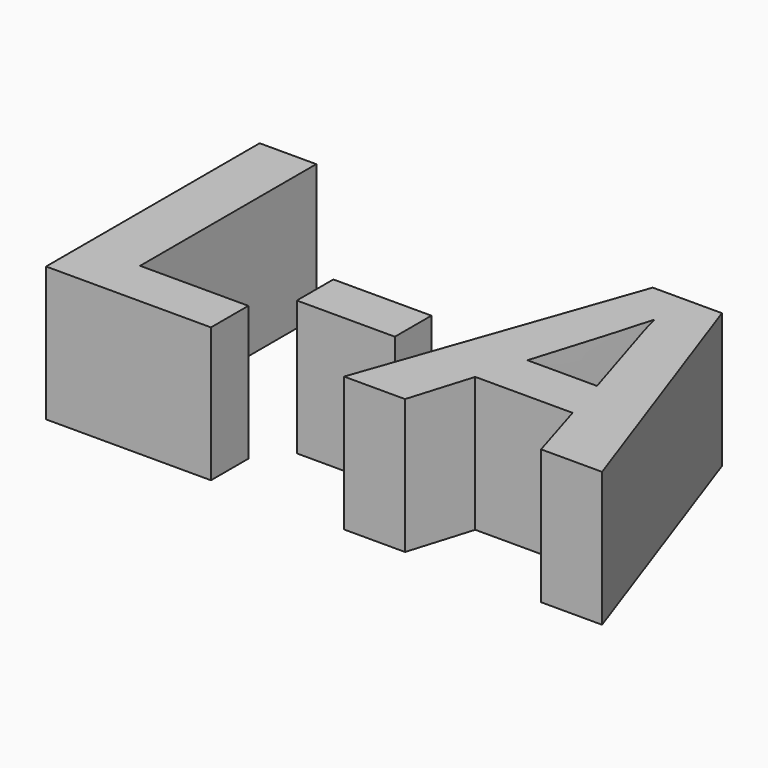
from build123d import *

# Parameters (mm, degrees)
F0_TEXT_SIZE = 70.5555555556
F1_DEPTH     = 25.4


# Not quite as in the source:
# - Text() gives the source's letters only with a copy of the font that has no kerning and outlines rounded to 1/6400 em; it was checked with that copy


with BuildPart() as f1:
    # F0 (on Top) → F1 (new body)
    with BuildSketch(Plane.XY):
        with Locations((-23.8532083449, -28.9006397721)):
            Text('L-A', F0_TEXT_SIZE, font='Open Sans', font_style=FontStyle.BOLD, text_align=(TextAlign.LEFT, TextAlign.BOTTOM))
    extrude(amount=F1_DEPTH)


solid = f1.part
